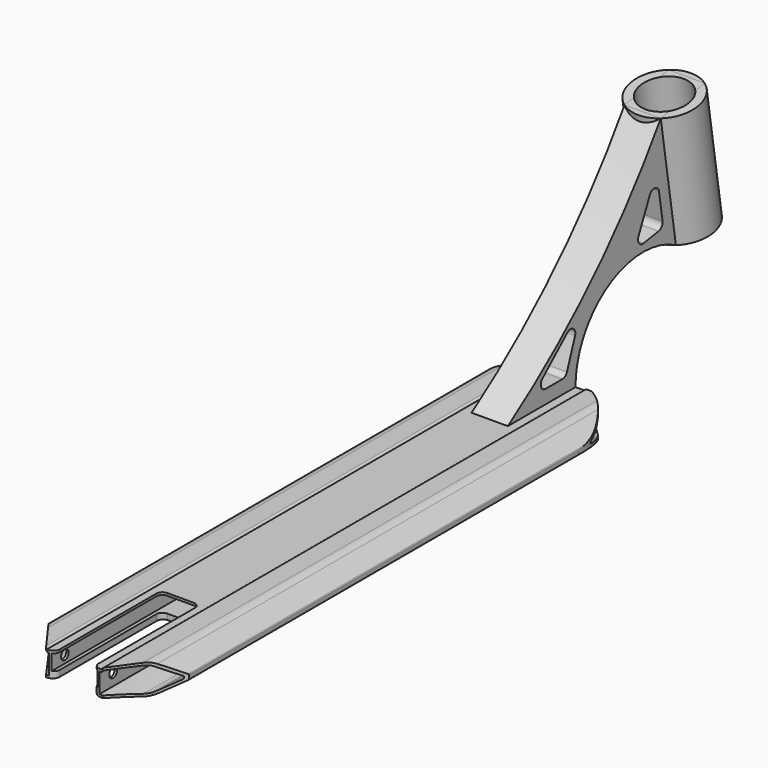
from build123d import *

# Parameters (mm, degrees)
F1_DEPTH    = 250
F2_W        = 38
F2_H        = 13
F3_DEPTH    = 250
F4_T1_DEPTH = 509.3674969976
F5_R        = 9
F6_R        = 1
F8_DEPTH    = 500.001
F10_DEPTH   = 15
F12_DEPTH   = 15
F13_F1_R    = 4.9999
F13_F2_R    = 4.9999
F13_F3_R    = 5
F13_F4_R    = 5
F13_F5_R    = 5
F13_F6_R    = 5
F15_DEPTH   = 15
F16_R       = 27.4590604355
F17_DEPTH   = 100
F19_D       = 40
F21_D       = 8
F23_DEPTH   = 72.5010001
F24_R       = 5


# Not quite as in the source:
# - a fillet or chamfer that OpenCascade refuses, or shapes differently, is made with other operations: its cross-section is extruded or revolved along the edge and cut away or added
# - a fillet or chamfer is up to 0.001 mm smaller than in the source, because OpenCascade refuses the exact size


with BuildPart() as f1:
    # F0 (on Front) → F1 (new body, symmetric)
    with BuildSketch(Plane.XZ):
        with BuildLine():
            Line((22.5, 11.3180404541), (-22.5, 11.3180404541))
            Line((-22.5, 11.3180404541), (-22.5, 12.6180404541))
            Line((-22.5, 12.6180404541), (-42.4624049573, 12.6180404541))
            Line((-42.4624049573, 12.6180404541), (-57.5, 0))
            Line((-57.5, 0), (-57.5, -4))
            Line((-57.5, -4), (-42.4624049573, -12.6819595459))
            ThreePointArc((-42.4624049573, -12.6819595459), (0, -8.1223447411), (42.4624049573, -12.6819595459))
            Line((42.4624049573, -12.6819595459), (57.5, -4))
            Line((57.5, -4), (57.5, 0))
            Line((57.5, 0), (42.4624049573, 12.6180404541))
            Line((42.4624049573, 12.6180404541), (22.5, 12.6180404541))
            Line((22.5, 12.6180404541), (22.5, 11.3180404541))
        make_face()
    extrude(amount=F1_DEPTH, both=True)

    # F2 (on Front) → F3 (cut, symmetric)
    with BuildSketch(Plane.XZ):
        with Locations((0, 2.8180404541)):
            Rectangle(F2_W, F2_H)
    extrude(amount=F3_DEPTH, both=True, mode=Mode.SUBTRACT)

    # F4: fillet of radius 2 on 2 edges, made by hand

    # F4_s2 → F4_t1 (cut)
    with BuildSketch(Plane.XZ.offset(-254.6837484988)):
        with BuildLine():
            ThreePointArc((-24.3734993995, 12.6180404541), (-23.2333239744, 12.2612081266), (-22.5, 11.3180404541))
            Line((-22.5, 11.3180404541), (-22.5, 12.6180404541))
            Line((-22.5, 12.6180404541), (-24.3734993995, 12.6180404541))
        make_face()
        with BuildLine():
            ThreePointArc((24.3734993995, 12.6180404541), (23.2333239744, 12.2612081266), (22.5, 11.3180404541))
            Line((22.5, 11.3180404541), (22.5, 12.6180404541))
            Line((22.5, 12.6180404541), (24.3734993995, 12.6180404541))
        make_face()
    extrude(amount=F4_T1_DEPTH, mode=Mode.SUBTRACT)

    # F5
    f5_edges = [f1.edges().sort_by_distance(p)[0] for p in [
        (-42.462405, 0, 12.61804),
        (-42.462405, 0, -12.68196),
        (42.462405, 0, 12.61804),
        (42.462405, 0, -12.68196),
    ]]
    fillet(f5_edges, radius=F5_R)

    # F6
    f6_edges = [f1.edges().sort_by_distance(p)[0] for p in [
        (57.5, 0, 0),
        (57.5, 0, -4),
        (-57.5, 0, 0),
        (-57.5, 0, -4),
    ]]
    fillet(f6_edges, radius=F6_R)

    # F7 (on face) → F8 (cut, through all)
    with BuildSketch(Plane.XZ.offset(250)):
        with BuildLine():
            ThreePointArc((-39.1866728489, 10.6180404541), (-41.5808138522, 10.1958887996), (-43.6861861167, 8.980351556))
            Line((-43.6861861167, 8.980351556), (-55.1427876097, -0.6328785313))
            ThreePointArc((-55.1427876097, -0.6328785313), (-55.406307787, -0.9763047127), (-55.5, -1.3989229745))
            Line((-55.5, -1.3989229745), (-55.5, -2.2679491924))
            ThreePointArc((-55.5, -2.2679491924), (-55.3660254038, -2.7679491924), (-55, -3.1339745962))
            Line((-55, -3.1339745962), (-44.4365005982, -9.2328138194))
            ThreePointArc((-44.4365005982, -9.2328138194), (-42.0740289831, -10.0775911234), (-39.5654216308, -10.0350472907))
            ThreePointArc((-39.5654216308, -10.0350472907), (-30.3154757647, -8.4101219575), (-21, -7.2168943421))
            Line((-21, -7.2168943421), (-21, 9.3180404541))
            Line((-21, 9.3180404541), (-22.5, 9.3180404541))
            ThreePointArc((-22.5, 9.3180404541), (-23.2333239744, 10.2612081266), (-24.3734993995, 10.6180404541))
            Line((-24.3734993995, 10.6180404541), (-39.1866728489, 10.6180404541))
        make_face()
        with BuildLine():
            ThreePointArc((39.5654216308, -10.0350472907), (42.0740289831, -10.0775911234), (44.4365005982, -9.2328138194))
            Line((44.4365005982, -9.2328138194), (55, -3.1339745962))
            ThreePointArc((55, -3.1339745962), (55.3660254038, -2.7679491924), (55.5, -2.2679491924))
            Line((55.5, -2.2679491924), (55.5, -1.3989229745))
            ThreePointArc((55.5, -1.3989229745), (55.406307787, -0.9763047127), (55.1427876097, -0.6328785313))
            Line((55.1427876097, -0.6328785313), (43.6861861167, 8.980351556))
            ThreePointArc((43.6861861167, 8.980351556), (41.5808138522, 10.1958887996), (39.1866728489, 10.6180404541))
            Line((39.1866728489, 10.6180404541), (24.3734993995, 10.6180404541))
            ThreePointArc((24.3734993995, 10.6180404541), (23.2333239744, 10.2612081266), (22.5, 9.3180404541))
            Line((22.5, 9.3180404541), (21, 9.3180404541))
            Line((21, 9.3180404541), (21, -7.2168943421))
            ThreePointArc((21, -7.2168943421), (30.3154757647, -8.4101219575), (39.5654216308, -10.0350472907))
        make_face()
    extrude(amount=-F8_DEPTH, mode=Mode.SUBTRACT)

    # F9 (on Top) → F10 (cut, symmetric)
    with BuildSketch(Plane.XY):
        with BuildLine():
            ThreePointArc((-57.5, 200), (0, 257.5), (57.5, 200))
            Line((57.5, 200), (57.5, 280))
            Line((57.5, 280), (-57.5, 280))
            Line((-57.5, 280), (-57.5, 200))
        make_face()
    extrude(amount=F10_DEPTH, both=True, mode=Mode.SUBTRACT)

    # F11 (on Top) → F12 (cut, symmetric)
    with BuildSketch(Plane.XY):
        Polygon((-23.3525011837, -250), (-57.5, -203), (-57.5, -257), (-57.5, -303), (57.5, -303), (57.5, -257), (57.5, -203), (23.3525011837, -250), (16, -250), (16, -140), (-16, -140), (-16, -250), align=None)
    extrude(amount=F12_DEPTH, both=True, mode=Mode.SUBTRACT)

    # F13: fillet of radius 5 on 8 edges, made by hand

    # F13_f1 (radius 5 in the source; OpenCascade refuses exactly that, so slightly less here)
    f13_f1_edges = [f1.edges().sort_by_distance(p)[0] for p in [
        (-16, -250, 10.3180404541),
    ]]
    fillet(f13_f1_edges, radius=F13_F1_R)

    # F13_f2 (radius 5 in the source; OpenCascade refuses exactly that, so slightly less here)
    f13_f2_edges = [f1.edges().sort_by_distance(p)[0] for p in [
        (16, -250, -6.2226657884),
    ]]
    fillet(f13_f2_edges, radius=F13_F2_R)

    # F13_f3
    f13_f3_edges = [f1.edges().sort_by_distance(p)[0] for p in [
        (16, -140, 10.3180404541),
    ]]
    fillet(f13_f3_edges, radius=F13_F3_R)

    # F13_f4
    f13_f4_edges = [f1.edges().sort_by_distance(p)[0] for p in [
        (-16, -140, 10.3180404541),
    ]]
    fillet(f13_f4_edges, radius=F13_F4_R)

    # F13_f5
    f13_f5_edges = [f1.edges().sort_by_distance(p)[0] for p in [
        (-16, -140, -6.2226657884),
    ]]
    fillet(f13_f5_edges, radius=F13_F5_R)

    # F13_f6
    f13_f6_edges = [f1.edges().sort_by_distance(p)[0] for p in [
        (16, -140, -6.2226657884),
    ]]
    fillet(f13_f6_edges, radius=F13_F6_R)

    # F14 (on Right) → F15 (join, symmetric)
    with BuildSketch(Plane.YZ):
        with BuildLine():
            ThreePointArc((338.2791760003, 171.3180404541), (267.4111014354, 83.1354883866), (180, 11.3180404541))
            Line((180, 11.3180404541), (250, 11.3180404541))
            ThreePointArc((250, 11.3180404541), (284.465394158, 71.6280047026), (353.9226225043, 72.5492063946))
            Line((353.9226225043, 72.5492063946), (399.3562861717, 79.7451917865))
            Line((399.3562861717, 79.7451917865), (383.7128396676, 178.514025846))
            Line((383.7128396676, 178.514025846), (338.2791760003, 171.3180404541))
        make_face()
    extrude(amount=F15_DEPTH, both=True)

    # F16 (on face) → F17 (join, through all)
    with BuildSketch(Plane(origin=(0, -18.1918123025, 114.8585824799), x_dir=(1, 0, 0), z_dir=(0, -0.156434465, 0.9876883406))):
        with Locations((0, 383.9144440118)):
            Circle(F16_R)
    extrude(amount=-F17_DEPTH)

    # F19 (through all)
    with Locations(Plane(origin=(0, -18.1918123025, 114.8585824799), x_dir=(1, 0, 0), z_dir=(0, -0.156434465, 0.9876883406))):
        with Locations((0, 383.9144440118)):
            Hole(F19_D / 2)

    # F21 (through all)
    with Locations(Plane.YZ.offset(21)):
        with Locations((-236, 2.7831056579)):
            Hole(F21_D / 2)

    # F22 (on face) → F23 (cut, through all)
    with BuildSketch(Plane.YZ.offset(15)):
        Polygon((333.8774988707, 135.1846038829), (311.2863995797, 86.0455946049), (340.9170497975, 90.7386285561), align=None)
        Polygon((240, 22.6180404541), (256.378660542, 67.6180404541), (206, 22.6180404541), align=None)
    extrude(amount=-F23_DEPTH, mode=Mode.SUBTRACT)

    # F24
    f24_edges = [f1.edges().sort_by_distance(p)[0] for p in [
        (0, 333.877499, 135.184604),
        (0, 340.91705, 90.738629),
        (0, 311.2864, 86.045595),
        (0, 256.378661, 67.61804),
        (0, 240, 22.61804),
        (0, 206, 22.61804),
    ]]
    fillet(f24_edges, radius=F24_R)


solid = f1.part
